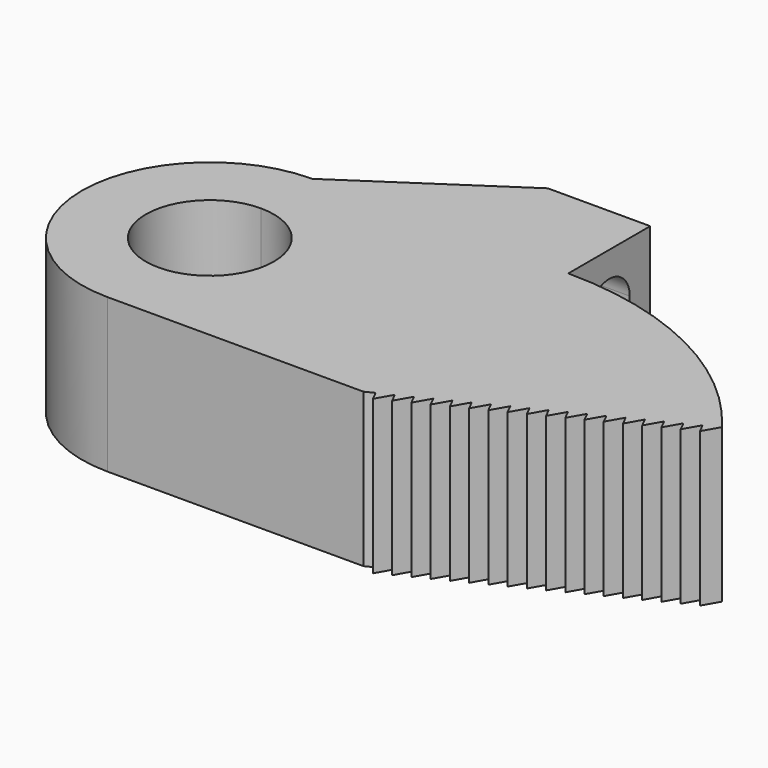
from build123d import *

# Parameters (mm, degrees)
F1_DEPTH = 7.62
F3_DEPTH = 7.62
F4_W     = 2.54
F4_H     = 2.54
F5_DEPTH = 25.4
F6_R     = 1.26999


# Not quite as in the source:
# - a fillet or chamfer is up to 0.001 mm smaller than in the source, because OpenCascade refuses the exact size


with BuildPart() as f1:
    # F0 (on Top) → F1 (new body)
    with BuildSketch(Plane.XY):
        with BuildLine():
            Line((-12.7, -6.35), (-12.7, 0))
            Line((-12.7, 0), (-19.05, 0))
            ThreePointArc((-19.05, 0), (-20.9098719395, -4.4901280605), (-25.4, -6.35))
            Line((-25.4, -6.35), (-12.7, -6.35))
        make_face()
        with BuildLine():
            Line((-12.7, 6.35), (-12.7, 0))
            Line((-12.7, 0), (-2.2980148465, 0))
            Line((-2.2980148465, 0), (-1.3816523133, 0.5641126772))
            Line((-1.3816523133, 0.5641126772), (0, 0))
            ThreePointArc((0, 0), (-5.6004841714, 4.6740316571), (-12.7, 6.35))
        make_face()
        with BuildLine():
            Line((-19.05, 0), (-12.7, 0))
            Line((-12.7, 0), (-12.7, 6.35))
            Line((-12.7, 6.35), (-25.4, 6.35))
            ThreePointArc((-25.4, 6.35), (-20.9098719395, 4.4901280605), (-19.05, 0))
        make_face()
        Polygon((-2.2980148465, 0), (-12.7, 0), (-12.7, -6.35), (-12.2375346417, -6.1187673209), align=None)
        with BuildLine():
            ThreePointArc((-25.4, -6.35), (-20.9098719395, -4.4901280605), (-19.05, 0))
            Line((-19.05, 0), (-22.225, 0))
            ThreePointArc((-22.225, 0), (-23.1549359697, -2.2450640303), (-25.4, -3.175))
            Line((-25.4, -3.175), (-25.4, -6.35))
        make_face()
        with BuildLine():
            Line((-22.225, 0), (-19.05, 0))
            ThreePointArc((-19.05, 0), (-20.9098719395, 4.4901280605), (-25.4, 6.35))
            Line((-25.4, 6.35), (-25.4, 3.175))
            ThreePointArc((-25.4, 3.175), (-23.1549359697, 2.2450640303), (-22.225, 0))
        make_face()
        Polygon((-1.3816523133, 0.5641126772), (-2.2980148465, 0), (0, 0), align=None)
        Polygon((0, 0), (-2.2980148465, 0), (-12.2375346417, -6.1187673209), (-0.6815535195, -0.3407767598), align=None)
        with BuildLine():
            Line((-25.4, 3.175), (-25.4, 6.35))
            ThreePointArc((-25.4, 6.35), (-31.75, 0), (-25.4, -6.35))
            Line((-25.4, -6.35), (-25.4, -3.175))
            ThreePointArc((-25.4, -3.175), (-28.575, 0), (-25.4, 3.175))
        make_face()
        Polygon((-0.454369013, -0.7951457728), (0, 0), (-0.6815535195, -0.3407767598), (-0.6815020435, -0.3408797119), align=None)
        Polygon((-0.6815535195, -0.3407767598), (-12.2375346417, -6.1187673209), (-12.2666181754, -6.1366711411), (-11.5850646558, -5.7958943813), (-11.3579903771, -6.2500430279), (-10.903621364, -5.4548972551), (-10.6765470852, -5.9090459018), (-10.2221780722, -5.113900129), (-9.9951037934, -5.5680487756), (-9.5407347804, -4.7729030028), (-9.3136605016, -5.2270516495), (-8.8592914886, -4.4319058767), (-8.6322172098, -4.8860545233), (-8.1778481968, -4.0909087505), (-7.950773918, -4.5450573971), (-7.496404905, -3.7499116243), (-7.2693306262, -4.204060271), (-6.8149616132, -3.4089144982), (-6.5878873344, -3.8630631448), (-6.1335183214, -3.067917372), (-5.9063852987, -3.5221834368), (-5.4520162857, -2.727037664), (-5.224883263, -3.1813037288), (-4.7705142499, -2.386157956), (-4.5433812273, -2.8404240208), (-4.0890122142, -2.045278248), (-3.8618791916, -2.4995443128), (-3.4075101785, -1.70439854), (-3.1803771559, -2.1586646048), (-2.7260081428, -1.363518832), (-2.4988751201, -1.8177848968), (-2.0445061071, -1.022639124), (-1.8173730844, -1.4769051888), (-1.3630040714, -0.681759416), (-1.1358710487, -1.1360254808), (-0.6815020357, -0.340879708), align=None)
        Polygon((-11.5850646558, -5.7958943813), (-12.2666181754, -6.1366711411), (-12.0394336689, -6.5910401541), align=None)
    extrude(amount=F1_DEPTH)

    # F2 (on face) → F3 (join)
    with BuildSketch(Plane.XY.offset(7.62)):
        Polygon((-25.4, 6.35), (-12.7, 6.35), (-12.7, 11.43), (-17.78, 11.43), align=None)
    extrude(amount=-F3_DEPTH)

    # F4 (on face) → F5 (cut)
    with BuildSketch(Plane.YZ.offset(-12.7)):
        with Locations((8.89, 2.54)):
            Rectangle(F4_W, F4_H)
        with Locations((8.89, 5.08)):
            Rectangle(F4_W, F4_H)
    extrude(amount=-F5_DEPTH, mode=Mode.SUBTRACT)

    # F6 (radius 1.27 in the source; OpenCascade refuses exactly that, so slightly less here)
    f6_edges = [f1.edges().sort_by_distance(p)[0] for p in [
        (-18.0975, 7.62, 1.27),
        (-18.0975, 7.62, 6.35),
        (-16.1925, 10.16, 6.35),
        (-16.1925, 10.16, 1.27),
    ]]
    fillet(f6_edges, radius=F6_R)


solid = f1.part
